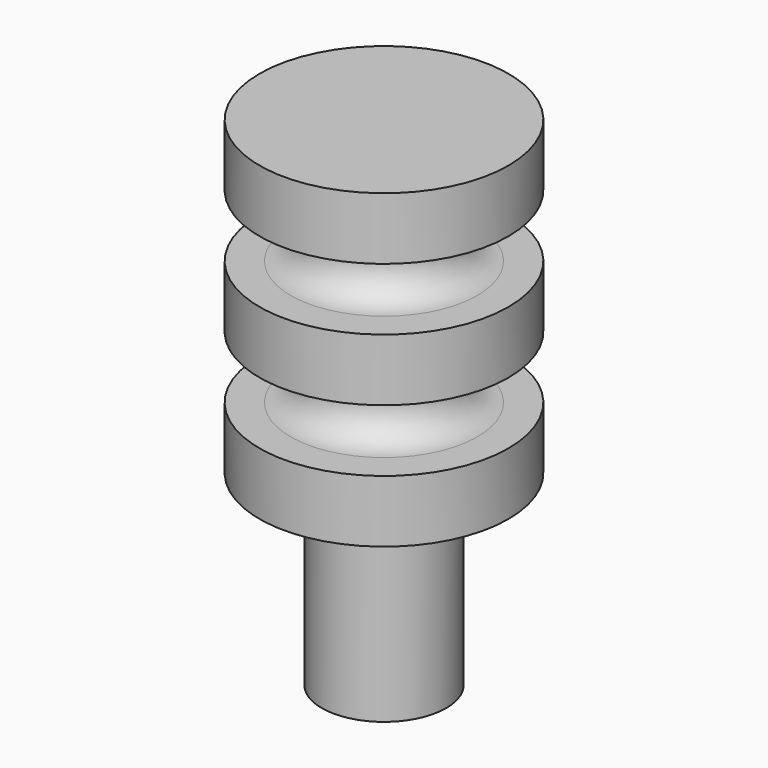
from build123d import *

# Parameters (mm, degrees)
F0_R     = 6.35
F0_R_2   = 3.175
F1_DEPTH = 15.875
F3_DEPTH = 9.525
F4_W     = 3.175
F4_H     = 3.175
F6_R     = 1.58749


# Not quite as in the source:
# - a fillet or chamfer is up to 0.001 mm smaller than in the source, because OpenCascade refuses the exact size


with BuildPart() as f1:
    # F0 (on Top) → F1 (new body)
    with BuildSketch(Plane.XY):
        Circle(F0_R)
        Circle(F0_R_2, mode=Mode.SUBTRACT)
        Circle(F0_R_2)
    extrude(amount=F1_DEPTH)

    # F0 (on Top) → F3 (join)
    with BuildSketch(Plane.XY):
        Circle(F0_R_2)
    extrude(amount=-F3_DEPTH)

    # F4 (on Right) → F5 (revolve, cut)
    with BuildSketch(Plane.YZ):
        with Locations((4.7625, 4.7625)):
            Rectangle(F4_W, F4_H)
        with Locations((4.7625, 11.1125)):
            Rectangle(F4_W, F4_H)
    revolve(axis=Axis((0, 0, -0.284396112), (0, 0, 1)), mode=Mode.SUBTRACT)

    # F6 (radius 1.5875 in the source; OpenCascade refuses exactly that, so slightly less here)
    f6_edges = [f1.edges().sort_by_distance(p)[0] for p in [
        (0, -3.175, 3.175),
        (0, -3.175, 6.35),
        (0, -3.175, 9.525),
        (0, -3.175, 12.7),
    ]]
    fillet(f6_edges, radius=F6_R)


solid = f1.part
